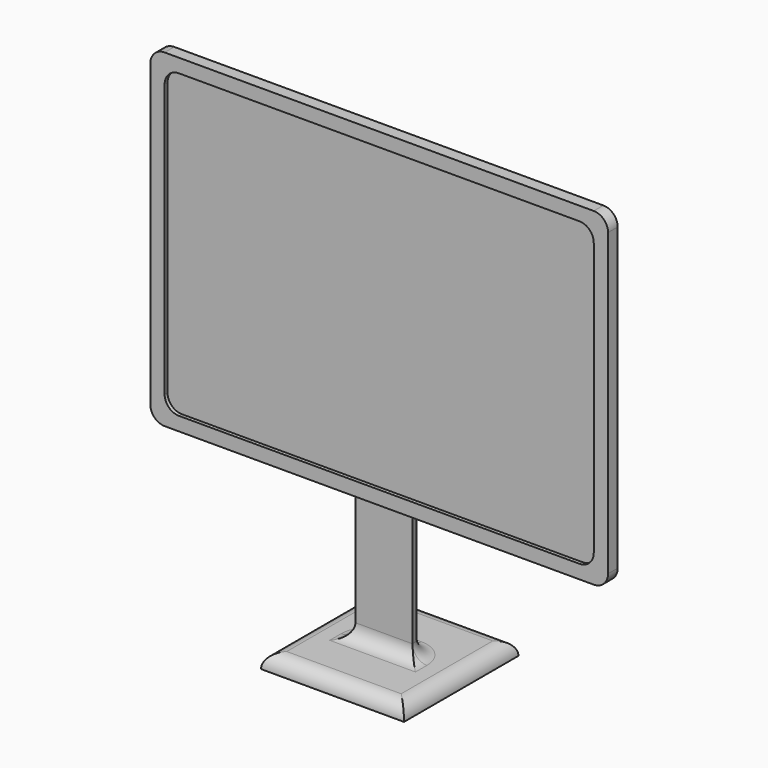
from build123d import *

# Parameters (mm, degrees)
F0_W     = 38.1
F0_H     = 26.7739508559
F1_DEPTH = 0.2116666666
F0_W_2   = 40.64
F0_H_2   = 29.21
F2_DEPTH = 0.5334
F3_W     = 5.08
F3_H     = 3.81
F3_H_2   = 11.481975428
F3_H_3   = 12.7
F4_DEPTH = 1.27
F5_W     = 12.7
F5_H     = 12.7
F6_DEPTH = 1.27
F7_R     = 1.26999
F7_2_R   = 1.26999
F8_R     = 1.27


# Not quite as in the source:
# - a fillet or chamfer is up to 0.001 mm smaller than in the source, because OpenCascade refuses the exact size


with BuildPart() as f1:
    # F0 (on Front) → F1 (new body)
    with BuildSketch(Plane.XZ):
        Rectangle(F0_W, F0_H)
    extrude(amount=F1_DEPTH)


with BuildPart() as f2:
    # F0 (on Front) → F2 (new body, symmetric)
    with BuildSketch(Plane.XZ):
        Rectangle(F0_W_2, F0_H_2)
        Rectangle(F0_W, F0_H, mode=Mode.SUBTRACT)
    extrude(amount=F2_DEPTH, both=True)

    # F7#2 (radius 1.27 in the source; OpenCascade refuses exactly that, so slightly less here)
    f7_2_edges = [f2.edges().sort_by_distance(p)[0] for p in [
        (-20.32, 0, -14.605),
        (20.32, 0, -14.605),
        (-20.32, 0, 14.605),
        (20.32, 0, 14.605),
    ]]
    fillet(f7_2_edges, radius=F7_2_R)

    # F8
    f8_edges = [f2.edges().sort_by_distance(p)[0] for p in [
        (-19.05, 0, 13.386975),
        (19.05, 0, 13.386975),
        (-19.05, 0, -13.386975),
        (19.05, 0, -13.386975),
    ]]
    fillet(f8_edges, radius=F8_R)


with BuildPart() as f4:
    # F3 (on face) → F4 (new body)
    with BuildSketch(Plane(origin=(0, 0, 0), x_dir=(-1, 0, 0), z_dir=(0, 1, 0))):
        Rectangle(F3_W, F3_H)
        with Locations((0, -7.645987714)):
            Rectangle(F3_W, F3_H_2)
        with Locations((0, -19.736975428)):
            Rectangle(F3_W, F3_H_3)
    extrude(amount=F4_DEPTH)

    # F5 (on face) → F6 (join)
    with BuildSketch(Plane(origin=(0, 0, -26.086975428), x_dir=(1, 0, 0), z_dir=(0, 0, -1))):
        with Locations((0, -0.635)):
            Rectangle(F5_W, F5_H)
    extrude(amount=F6_DEPTH)

    # F7 (radius 1.27 in the source; OpenCascade refuses exactly that, so slightly less here)
    f7_edges = [f4.edges().sort_by_distance(p)[0] for p in [
        (0, 0, -26.086975),
        (-2.54, 0.635, -26.086975),
        (2.54, 0.635, -26.086975),
        (0, 1.27, -26.086975),
        (0, 6.985, -26.086975),
        (6.35, 0.635, -26.086975),
        (0, -5.715, -26.086975),
        (-6.35, 0.635, -26.086975),
        (2.54, 1.27, -12.090988),
        (-2.54, 1.27, -12.090988),
        (0, 1.27, 1.905),
    ]]
    fillet(f7_edges, radius=F7_R)


solid = Compound([f1.part, f2.part, f4.part])
